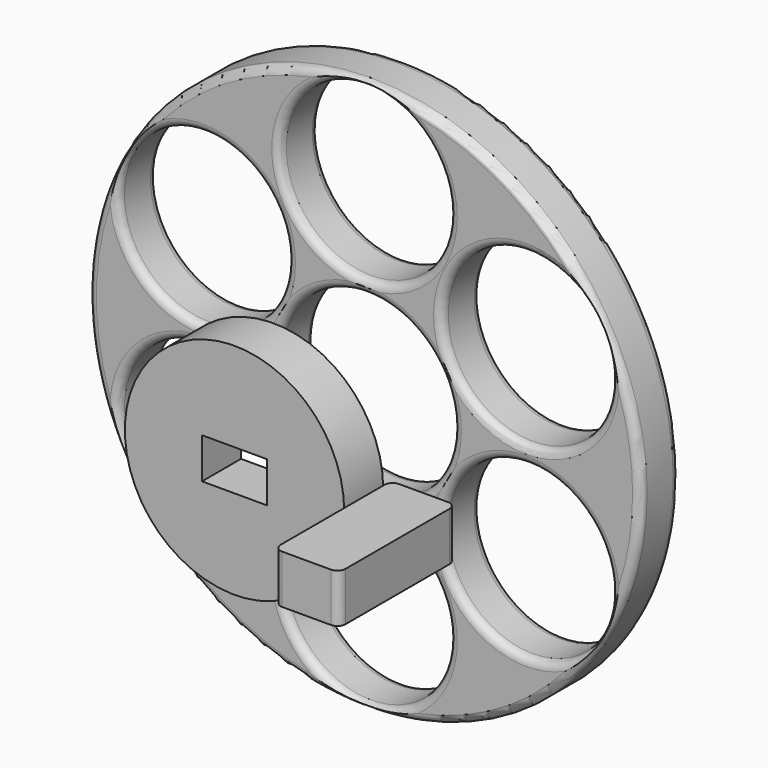
from build123d import *

# Parameters (mm, degrees)
F0_R     = 34
F0_R_2   = 10.425
F0_R_3   = 10.925
F1_DEPTH = 6
F4_DEPTH = 6
F6_START = 20
F5_R     = 13.5
F5_W     = 8
F5_H     = 5
F6_DEPTH = 6


# Not quite as in the source:
# - a fillet or chamfer that OpenCascade refuses, or shapes differently, is made with other operations: its cross-section is extruded or revolved along the edge and cut away or added
# - a feature names something its author has since deleted; it is built from what else it names


with BuildPart() as f1:
    # F0 (on Front) → F1 (new body)
    with BuildSketch(Plane.XZ):
        Circle(F0_R)
        with Locations((-19.918584287, -11.5)):
            Circle(F0_R_2, mode=Mode.SUBTRACT)
        with Locations((0, -23)):
            Circle(F0_R_2, mode=Mode.SUBTRACT)
        with Locations((19.918584287, -11.5)):
            Circle(F0_R_2, mode=Mode.SUBTRACT)
        with Locations((-19.918584287, 11.5)):
            Circle(F0_R_2, mode=Mode.SUBTRACT)
        Circle(F0_R_3, mode=Mode.SUBTRACT)
        with Locations((19.918584287, 11.5)):
            Circle(F0_R_2, mode=Mode.SUBTRACT)
        with Locations((0, 23)):
            Circle(F0_R_2, mode=Mode.SUBTRACT)
    extrude(amount=F1_DEPTH)

    # F2: fillet of radius 1 on 16 edges, made by hand

    # F2_s1 → F2_t2 (revolve, cut)
    with BuildSketch(Plane.XY):
        with BuildLine():
            ThreePointArc((34, -5), (33.7071067812, -5.7071067812), (33, -6))
            Line((33, -6), (34, -6))
            Line((34, -6), (34, -5))
        make_face()
    revolve(axis=Axis((0, -6, 0), (0, -1, 0)), mode=Mode.SUBTRACT)

    # F2_s3 → F2_t4 (revolve, cut)
    with BuildSketch(Plane.XY.offset(-11.5)):
        with BuildLine():
            ThreePointArc((-9.493584287, -5), (-9.2006910682, -5.7071067812), (-8.493584287, -6))
            Line((-8.493584287, -6), (-9.493584287, -6))
            Line((-9.493584287, -6), (-9.493584287, -5))
        make_face()
    revolve(axis=Axis((-19.918584287, -6, -11.5), (0, -1, 0)), mode=Mode.SUBTRACT)

    # F2_s5 → F2_t6 (revolve, cut)
    with BuildSketch(Plane.XY.offset(-23)):
        with BuildLine():
            ThreePointArc((10.425, -5), (10.7178932188, -5.7071067812), (11.425, -6))
            Line((11.425, -6), (10.425, -6))
            Line((10.425, -6), (10.425, -5))
        make_face()
    revolve(axis=Axis((0, -6, -23), (0, -1, 0)), mode=Mode.SUBTRACT)

    # F2_s7 → F2_t8 (revolve, cut)
    with BuildSketch(Plane.XY.offset(-11.5)):
        with BuildLine():
            ThreePointArc((30.343584287, -5), (30.6364775059, -5.7071067812), (31.343584287, -6))
            Line((31.343584287, -6), (30.343584287, -6))
            Line((30.343584287, -6), (30.343584287, -5))
        make_face()
    revolve(axis=Axis((19.918584287, -6, -11.5), (0, -1, 0)), mode=Mode.SUBTRACT)

    # F2_s9 → F2_t10 (revolve, cut)
    with BuildSketch(Plane.XY.offset(11.5)):
        with BuildLine():
            ThreePointArc((-9.493584287, -5), (-9.2006910682, -5.7071067812), (-8.493584287, -6))
            Line((-8.493584287, -6), (-9.493584287, -6))
            Line((-9.493584287, -6), (-9.493584287, -5))
        make_face()
    revolve(axis=Axis((-19.918584287, -6, 11.5), (0, -1, 0)), mode=Mode.SUBTRACT)

    # F2_s11 → F2_t12 (revolve, cut)
    with BuildSketch(Plane.XY):
        with BuildLine():
            ThreePointArc((10.925, -5), (11.2178932188, -5.7071067812), (11.925, -6))
            Line((11.925, -6), (10.925, -6))
            Line((10.925, -6), (10.925, -5))
        make_face()
    revolve(axis=Axis((0, -6, 0), (0, -1, 0)), mode=Mode.SUBTRACT)

    # F2_s13 → F2_t14 (revolve, cut)
    with BuildSketch(Plane.XY.offset(11.5)):
        with BuildLine():
            ThreePointArc((30.343584287, -5), (30.6364775059, -5.7071067812), (31.343584287, -6))
            Line((31.343584287, -6), (30.343584287, -6))
            Line((30.343584287, -6), (30.343584287, -5))
        make_face()
    revolve(axis=Axis((19.918584287, -6, 11.5), (0, -1, 0)), mode=Mode.SUBTRACT)

    # F2_s15 → F2_t16 (revolve, cut)
    with BuildSketch(Plane.XY.offset(23)):
        with BuildLine():
            ThreePointArc((10.425, -5), (10.7178932188, -5.7071067812), (11.425, -6))
            Line((11.425, -6), (10.425, -6))
            Line((10.425, -6), (10.425, -5))
        make_face()
    revolve(axis=Axis((0, -6, 23), (0, -1, 0)), mode=Mode.SUBTRACT)

    # F2_s17 → F2_t18 (revolve, cut)
    with BuildSketch(Plane.XY):
        with BuildLine():
            ThreePointArc((34, -1), (33.7071067812, -0.2928932188), (33, 0))
            Line((33, 0), (34, 0))
            Line((34, 0), (34, -1))
        make_face()
    revolve(axis=Axis((0, 0, 0), (0, -1, 0)), mode=Mode.SUBTRACT)

    # F2_s19 → F2_t20 (revolve, cut)
    with BuildSketch(Plane.XY.offset(-11.5)):
        with BuildLine():
            ThreePointArc((-9.493584287, -1), (-9.2006910682, -0.2928932188), (-8.493584287, 0))
            Line((-8.493584287, 0), (-9.493584287, 0))
            Line((-9.493584287, 0), (-9.493584287, -1))
        make_face()
    revolve(axis=Axis((-19.918584287, 0, -11.5), (0, -1, 0)), mode=Mode.SUBTRACT)

    # F2_s21 → F2_t22 (revolve, cut)
    with BuildSketch(Plane.XY.offset(-23)):
        with BuildLine():
            ThreePointArc((10.425, -1), (10.7178932188, -0.2928932188), (11.425, 0))
            Line((11.425, 0), (10.425, 0))
            Line((10.425, 0), (10.425, -1))
        make_face()
    revolve(axis=Axis((0, 0, -23), (0, -1, 0)), mode=Mode.SUBTRACT)

    # F2_s23 → F2_t24 (revolve, cut)
    with BuildSketch(Plane.XY.offset(-11.5)):
        with BuildLine():
            ThreePointArc((30.343584287, -1), (30.6364775059, -0.2928932188), (31.343584287, 0))
            Line((31.343584287, 0), (30.343584287, 0))
            Line((30.343584287, 0), (30.343584287, -1))
        make_face()
    revolve(axis=Axis((19.918584287, 0, -11.5), (0, -1, 0)), mode=Mode.SUBTRACT)

    # F2_s25 → F2_t26 (revolve, cut)
    with BuildSketch(Plane.XY.offset(11.5)):
        with BuildLine():
            ThreePointArc((-9.493584287, -1), (-9.2006910682, -0.2928932188), (-8.493584287, 0))
            Line((-8.493584287, 0), (-9.493584287, 0))
            Line((-9.493584287, 0), (-9.493584287, -1))
        make_face()
    revolve(axis=Axis((-19.918584287, 0, 11.5), (0, -1, 0)), mode=Mode.SUBTRACT)

    # F2_s27 → F2_t28 (revolve, cut)
    with BuildSketch(Plane.XY):
        with BuildLine():
            ThreePointArc((10.925, -1), (11.2178932188, -0.2928932188), (11.925, 0))
            Line((11.925, 0), (10.925, 0))
            Line((10.925, 0), (10.925, -1))
        make_face()
    revolve(axis=Axis((0, 0, 0), (0, -1, 0)), mode=Mode.SUBTRACT)

    # F2_s29 → F2_t30 (revolve, cut)
    with BuildSketch(Plane.XY.offset(11.5)):
        with BuildLine():
            ThreePointArc((30.343584287, -1), (30.6364775059, -0.2928932188), (31.343584287, 0))
            Line((31.343584287, 0), (30.343584287, 0))
            Line((30.343584287, 0), (30.343584287, -1))
        make_face()
    revolve(axis=Axis((19.918584287, 0, 11.5), (0, -1, 0)), mode=Mode.SUBTRACT)

    # F2_s31 → F2_t32 (revolve, cut)
    with BuildSketch(Plane.XY.offset(23)):
        with BuildLine():
            ThreePointArc((10.425, -1), (10.7178932188, -0.2928932188), (11.425, 0))
            Line((11.425, 0), (10.425, 0))
            Line((10.425, 0), (10.425, -1))
        make_face()
    revolve(axis=Axis((0, 0, 23), (0, -1, 0)), mode=Mode.SUBTRACT)


with BuildPart() as f4:
    # F3 (on Top) → F4 (new body)
    with BuildSketch(Plane.XY):
        with BuildLine():
            Line((27.347636193, -27.3550294042), (21.347636193, -27.3550294042))
            ThreePointArc((21.347636193, -27.3550294042), (20.6405294119, -27.647922623), (20.347636193, -28.3550294042))
            Line((20.347636193, -28.3550294042), (20.347636193, -44.3550294042))
            ThreePointArc((20.347636193, -44.3550294042), (20.6405294119, -45.0621361853), (21.347636193, -45.3550294042))
            Line((21.347636193, -45.3550294042), (27.347636193, -45.3550294042))
            ThreePointArc((27.347636193, -45.3550294042), (28.0547429742, -45.0621361853), (28.347636193, -44.3550294042))
            Line((28.347636193, -44.3550294042), (28.347636193, -28.3550294042))
            ThreePointArc((28.347636193, -28.3550294042), (28.0547429742, -27.647922623), (27.347636193, -27.3550294042))
        make_face()
    extrude(amount=F4_DEPTH)


with BuildPart() as f6:
    # F5 (on Front) → F6 (new body)
    with BuildSketch(Plane.XZ.offset(F6_START)):
        Circle(F5_R)
        Rectangle(F5_W, F5_H, mode=Mode.SUBTRACT)
    extrude(amount=F6_DEPTH)


solid = Compound([f1.part, f4.part, f6.part])
